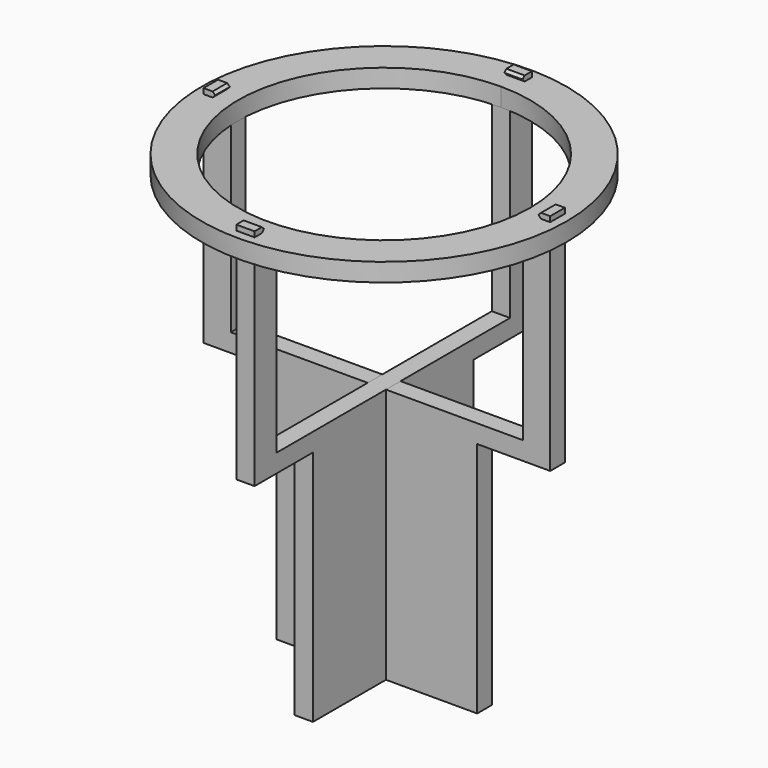
from build123d import *

# Parameters (mm, degrees)
F1_DEPTH = 3.175
F3_DEPTH = 3.175
F4_R     = 63.5
F4_W     = 6.35
F4_H     = 3.175
F4_W_2   = 3.175
F4_H_2   = 6.35
F5_DEPTH = 6.35


# Not quite as in the source:
# - a feature names something its author has since deleted; it is built from what else it names


with BuildPart() as f1:
    # F0 (on Front) → F1 (new body, symmetric)
    with BuildSketch(Plane.XZ):
        Polygon((-34.925, -82.55), (0, -82.55), (34.925, -82.55), (34.925, 0), (60.325, 0), (60.325, 69.85), (57.15, 69.85), (50.8, 69.85), (50.8, 6.35), (3.175, 6.35), (3.175, -38.1), (-3.175, -38.1), (-3.175, 6.35), (-50.8, 6.35), (-50.8, 69.85), (-57.15, 69.85), (-60.325, 69.85), (-60.325, 0), (-34.925, 0), align=None)
        Polygon((-60.325, 78.0568867745), (-60.325, 69.85), (-57.15, 69.85), (-57.15, 76.2), (-56.2234869578, 77.1882823867), (-57.15, 78.0568867745), align=None)
        Polygon((57.15, 69.85), (60.325, 69.85), (60.325, 78.0568867745), (57.15, 78.0568867745), (56.2234869578, 77.1882823867), (57.15, 76.2), align=None)
    extrude(amount=F1_DEPTH, both=True)


with BuildPart() as f3:
    # F2 (on Right) → F3 (new body, symmetric)
    with BuildSketch(Plane.YZ):
        Polygon((3.175, -38.1), (3.175, -82.55), (34.925, -82.55), (34.925, 0), (60.325, 0), (60.325, 69.85), (57.15, 69.85), (50.8, 69.85), (50.8, 6.35), (3.175, 6.35), (-3.175, 6.35), (-50.8, 6.35), (-50.8, 69.85), (-57.15, 69.85), (-60.325, 69.85), (-60.325, 0), (-34.925, 0), (-34.925, -82.55), (-3.175, -82.55), (-3.175, -38.1), (0, -38.1), align=None)
        Polygon((57.15, 69.85), (60.325, 69.85), (60.325, 78.0568867745), (57.15, 78.0568867745), (56.2234869578, 77.1882823867), (57.15, 76.2), align=None)
        Polygon((-60.325, 78.0568867745), (-60.325, 69.85), (-57.15, 69.85), (-57.15, 76.2), (-56.2234869578, 77.1882823867), (-57.15, 78.0568867745), align=None)
    extrude(amount=F3_DEPTH, both=True)


with BuildPart() as f5:
    # F4 (on face) → F5 (new body)
    with BuildSketch(Plane.XY.offset(69.85)):
        Circle(F4_R)
        with Locations((0, -58.7375)):
            Rectangle(F4_W, F4_H, mode=Mode.SUBTRACT)
        with Locations((-58.7375, 0)):
            Rectangle(F4_W_2, F4_H_2, mode=Mode.SUBTRACT)
        with BuildLine():
            ThreePointArc((-6.22e-08, 50.8), (35.9210244623, 35.9210245063), (50.8, 0))
            ThreePointArc((50.8, 0), (-35.9210244623, -35.9210245063), (-6.22e-08, 50.8))
        make_face(mode=Mode.SUBTRACT)
        with Locations((58.7375, 0)):
            Rectangle(F4_W_2, F4_H_2, mode=Mode.SUBTRACT)
        Polygon((3.175, 50.8), (-6.22e-08, 50.8), (-3.175, 50.8), (-3.175, 57.15), (-3.175, 60.325), (3.175, 60.325), (3.175, 57.15), align=None, mode=Mode.SUBTRACT)
        Polygon((-3.175, 50.8), (-6.22e-08, 50.8), (3.175, 50.8), (3.175, 57.15), (-3.175, 57.15), align=None)
    extrude(amount=F5_DEPTH)


solid = Compound([f1.part, f3.part, f5.part])
